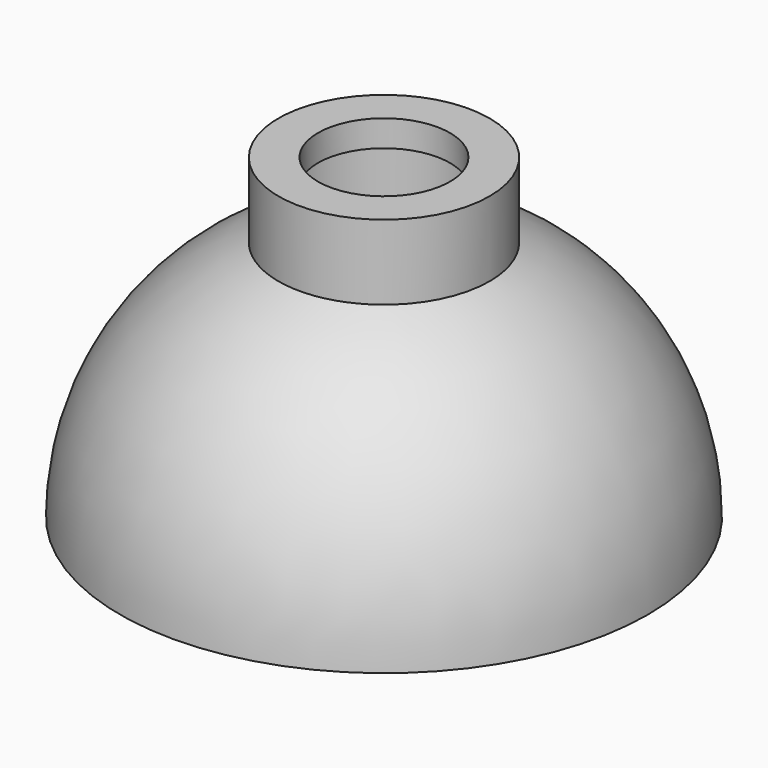
from build123d import *

# Parameters (mm, degrees)
F1_R     = 25.4
F1_R_2   = 10.16
F2_DEPTH = 25.4
F3_R     = 25.39999
F4_DEPTH = 30.48
F7_D     = 16.51
F8_DEPTH = 7.62
F9_START = 27.94
F9_DEPTH = 2.54


# Not quite as in the source:
# - a variable given as a bare number and used for a length is read in inches; the dataset says mm whatever the document's units were
# - a fillet or chamfer is up to 0.001 mm smaller than in the source, because OpenCascade refuses the exact size


with BuildPart() as f2:
    # F1 (on Top) → F2 (new body)
    with BuildSketch(Plane.XY):
        Circle(F1_R)
        Circle(F1_R_2, mode=Mode.SUBTRACT)
        Circle(F1_R_2)
    extrude(amount=F2_DEPTH)

    # F3 (radius 25.4 in the source; OpenCascade refuses exactly that, so slightly less here)
    f3_edges = [f2.edges().sort_by_distance(p)[0] for p in [
        (-25.4, 0, 25.4),
    ]]
    fillet(f3_edges, radius=F3_R)

    # F1 (on Top) → F4 (join)
    with BuildSketch(Plane.XY):
        Circle(F1_R_2)
    extrude(amount=F4_DEPTH)

    # F7 (through all)
    with Locations(Plane(origin=(0, 0, 0), x_dir=(1, 0, 0), z_dir=(0, 0, -1))):
        with Locations((0, 0)):
            Hole(F7_D / 2)

    # F6 (on face) → F8 (join)
    with BuildSketch(Plane.XY):
        with BuildLine():
            ThreePointArc((-6.35, 0), (0, -6.35), (6.35, 0))
            Line((6.35, 0), (3.175, 0))
            ThreePointArc((3.175, 0), (0, -3.175), (-3.175, 0))
            Line((-3.175, 0), (-6.35, 0))
        make_face()
        with BuildLine():
            Line((3.175, 0), (6.35, 0))
            ThreePointArc((6.35, 0), (0, 6.35), (-6.35, 0))
            Line((-6.35, 0), (-3.175, 0))
            ThreePointArc((-3.175, 0), (0, 3.175), (3.175, 0))
        make_face()
        with BuildLine():
            Line((8.255, 0), (6.35, 0))
            ThreePointArc((6.35, 0), (0, -6.35), (-6.35, 0))
            Line((-6.35, 0), (-8.255, 0))
            ThreePointArc((-8.255, 0), (0, -8.255), (8.255, 0))
        make_face()
        with BuildLine():
            ThreePointArc((-6.35, 0), (0, 6.35), (6.35, 0))
            Line((6.35, 0), (8.255, 0))
            ThreePointArc((8.255, 0), (0, 8.255), (-8.255, 0))
            Line((-8.255, 0), (-6.35, 0))
        make_face()
    extrude(amount=F8_DEPTH)

    # F6 (on face) → F9 (join)
    with BuildSketch(Plane.XY.offset(F9_START)):
        with BuildLine():
            Line((8.255, 0), (6.35, 0))
            ThreePointArc((6.35, 0), (0, -6.35), (-6.35, 0))
            Line((-6.35, 0), (-8.255, 0))
            ThreePointArc((-8.255, 0), (0, -8.255), (8.255, 0))
        make_face()
        with BuildLine():
            ThreePointArc((-6.35, 0), (0, 6.35), (6.35, 0))
            Line((6.35, 0), (8.255, 0))
            ThreePointArc((8.255, 0), (0, 8.255), (-8.255, 0))
            Line((-8.255, 0), (-6.35, 0))
        make_face()
    extrude(amount=F9_DEPTH)


solid = f2.part
